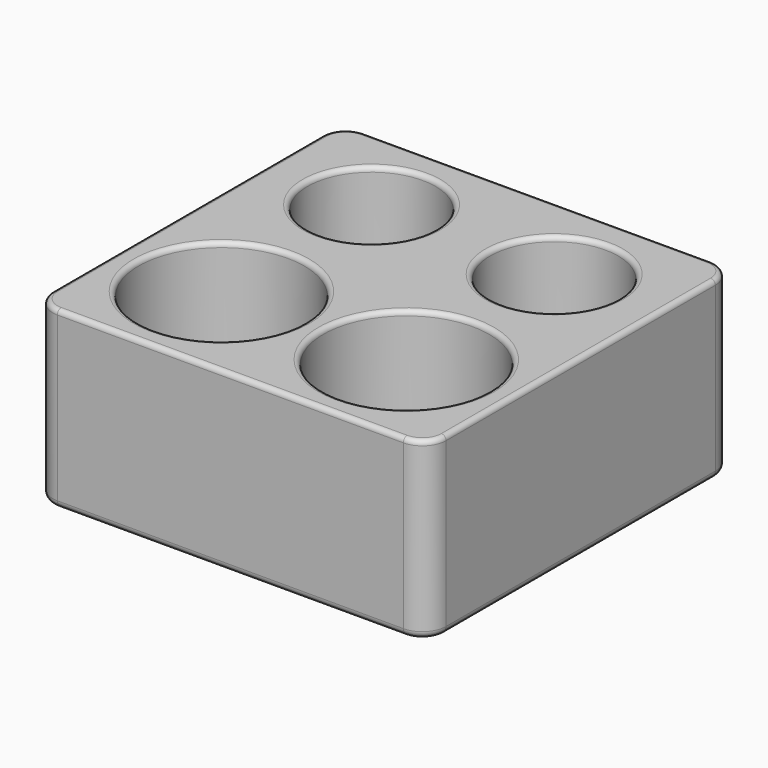
from build123d import *

# Parameters (mm, degrees)
F0_W         = 83
F0_H         = 81
F0_R         = 17.5
F0_R_2       = 13.5
F1_DEPTH     = 36
F2_R         = 1
F3_W         = 83
F3_H         = 81
F4_DEPTH     = 1
F5_T1_DEPTH  = 49.5
F5_T4_ANGLE  = 90
F5_T6_ANGLE  = 90
F5_T8_ANGLE  = 90
F5_T10_ANGLE = 90
F6_R         = 1.5


# Not quite as in the source:
# - a fillet or chamfer that OpenCascade refuses, or shapes differently, is made with other operations: its cross-section is extruded or revolved along the edge and cut away or added
# - a feature names something its author has since deleted; it is built from what else it names


with BuildPart() as f1:
    # F0 (on Top) → F1 (new body)
    with BuildSketch(Plane.XY):
        with Locations((-3, 18.5)):
            Rectangle(F0_W, F0_H)
        with Locations((-22.5, 0)):
            Circle(F0_R, mode=Mode.SUBTRACT)
        with Locations((16.5, 0)):
            Circle(F0_R, mode=Mode.SUBTRACT)
        with Locations((-22.5, 39.5840890706)):
            Circle(F0_R_2, mode=Mode.SUBTRACT)
        with Locations((16.5, 39)):
            Circle(F0_R_2, mode=Mode.SUBTRACT)
    extrude(amount=F1_DEPTH)

    # F2
    f2_edges = [f1.edges().sort_by_distance(p)[0] for p in [
        (-3, 59, 36),
        (-44.5, 18.5, 36),
        (-3, -22, 36),
        (38.5, 18.5, 36),
        (-40, 0, 36),
        (-1, 0, 36),
        (-36, 39.584089, 36),
        (3, 39, 36),
    ]]
    fillet(f2_edges, radius=F2_R)

    # F3 (on face) → F4 (join)
    with BuildSketch(Plane(origin=(0, 0, 0), x_dir=(1, 0, 0), z_dir=(0, 0, -1))):
        with Locations((-3, -18.5)):
            Rectangle(F3_W, F3_H)
    extrude(amount=F4_DEPTH)

    # F5: fillet of radius 5 on 4 edges, made by hand

    # F5_s2 → F5_t1 (cut)
    with BuildSketch(Plane.XY.offset(-13.5)):
        with BuildLine():
            ThreePointArc((-39.5, 59), (-43.0355339059, 57.5355339059), (-44.5, 54))
            Line((-44.5, 54), (-44.5, 59))
            Line((-44.5, 59), (-39.5, 59))
        make_face()
        with BuildLine():
            ThreePointArc((-39.5, -22), (-43.0355339059, -20.5355339059), (-44.5, -17))
            Line((-44.5, -17), (-44.5, -22))
            Line((-44.5, -22), (-39.5, -22))
        make_face()
        with BuildLine():
            ThreePointArc((33.5, -22), (37.0355339059, -20.5355339059), (38.5, -17))
            Line((38.5, -17), (38.5, -22))
            Line((38.5, -22), (33.5, -22))
        make_face()
        with BuildLine():
            ThreePointArc((33.5, 59), (37.0355339059, 57.5355339059), (38.5, 54))
            Line((38.5, 54), (38.5, 59))
            Line((38.5, 59), (33.5, 59))
        make_face()
    extrude(amount=F5_T1_DEPTH, mode=Mode.SUBTRACT)

    # F5_s3 → F5_t4 (revolve, cut)
    with BuildSketch(Plane.XZ.offset(-54)):
        with BuildLine():
            ThreePointArc((37.5, 36), (38.2071067812, 35.7071067812), (38.5, 35))
            Line((38.5, 35), (38.5, 36))
            Line((38.5, 36), (37.5, 36))
        make_face()
    revolve(axis=Axis((33.5, 54, 36), (0, 0, 1)), revolution_arc=F5_T4_ANGLE, mode=Mode.SUBTRACT)

    # F5_s5 → F5_t6 (revolve, cut)
    with BuildSketch(Plane.YZ.offset(33.5)):
        with BuildLine():
            ThreePointArc((-21, 36), (-21.7071067812, 35.7071067812), (-22, 35))
            Line((-22, 35), (-22, 36))
            Line((-22, 36), (-21, 36))
        make_face()
    revolve(axis=Axis((33.5, -17, 36), (0, 0, 1)), revolution_arc=F5_T6_ANGLE, mode=Mode.SUBTRACT)

    # F5_s7 → F5_t8 (revolve, cut)
    with BuildSketch(Plane.XZ.offset(17)):
        with BuildLine():
            ThreePointArc((-43.5, 36), (-44.2071067812, 35.7071067812), (-44.5, 35))
            Line((-44.5, 35), (-44.5, 36))
            Line((-44.5, 36), (-43.5, 36))
        make_face()
    revolve(axis=Axis((-39.5, -17, 36), (0, 0, 1)), revolution_arc=F5_T8_ANGLE, mode=Mode.SUBTRACT)

    # F5_s9 → F5_t10 (revolve, cut)
    with BuildSketch(Plane.YZ.offset(-39.5)):
        with BuildLine():
            ThreePointArc((58, 36), (58.7071067812, 35.7071067812), (59, 35))
            Line((59, 35), (59, 36))
            Line((59, 36), (58, 36))
        make_face()
    revolve(axis=Axis((-39.5, 54, 36), (0, 0, 1)), revolution_arc=F5_T10_ANGLE, mode=Mode.SUBTRACT)

    # F6
    f6_edges = [f1.edges().sort_by_distance(p)[0] for p in [
        (37.035534, -20.535534, -1),
        (38.5, 18.5, -1),
        (37.035534, 57.535534, -1),
        (-3, 59, -1),
        (-43.035534, 57.535534, -1),
        (-44.5, 18.5, -1),
        (-43.035534, -20.535534, -1),
        (-3, -22, -1),
    ]]
    fillet(f6_edges, radius=F6_R)


solid = f1.part
